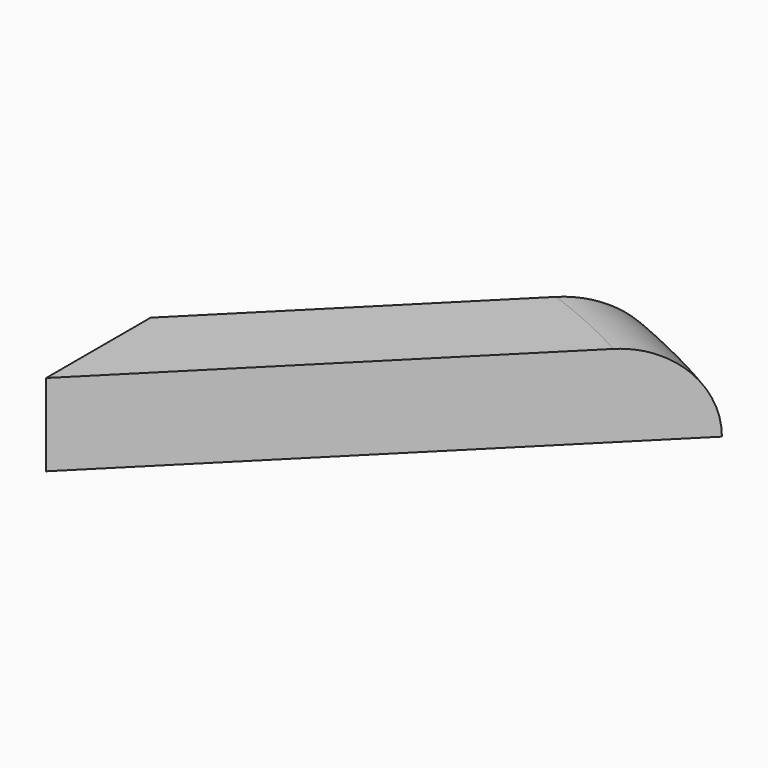
from build123d import *

# Parameters (mm, degrees)
F2_DEPTH = 25.4
F3_R     = 25.39999


# Not quite as in the source:
# - a fillet or chamfer is up to 0.001 mm smaller than in the source, because OpenCascade refuses the exact size


with BuildPart() as f2:
    # F1 (on face) → F2 (new body)
    with BuildSketch(Plane.XY):
        with BuildLine():
            Line((0, 121.2334576344), (0, 80.8223050896))
            Line((0, 80.8223050896), (116.1005682623, 196.9228733519))
            ThreePointArc((116.1005682623, 196.9228733519), (102.889252487, 204.1366251379), (89.2318353651, 210.4652929995))
            Line((89.2318353651, 210.4652929995), (0, 121.2334576344))
        make_face()
    extrude(amount=F2_DEPTH)

    # F3 (radius 25.4 in the source; OpenCascade refuses exactly that, so slightly less here)
    f3_edges = [f2.edges().sort_by_distance(p)[0] for p in [
        (102.889252, 204.136625, 25.4),
    ]]
    fillet(f3_edges, radius=F3_R)


solid = f2.part
